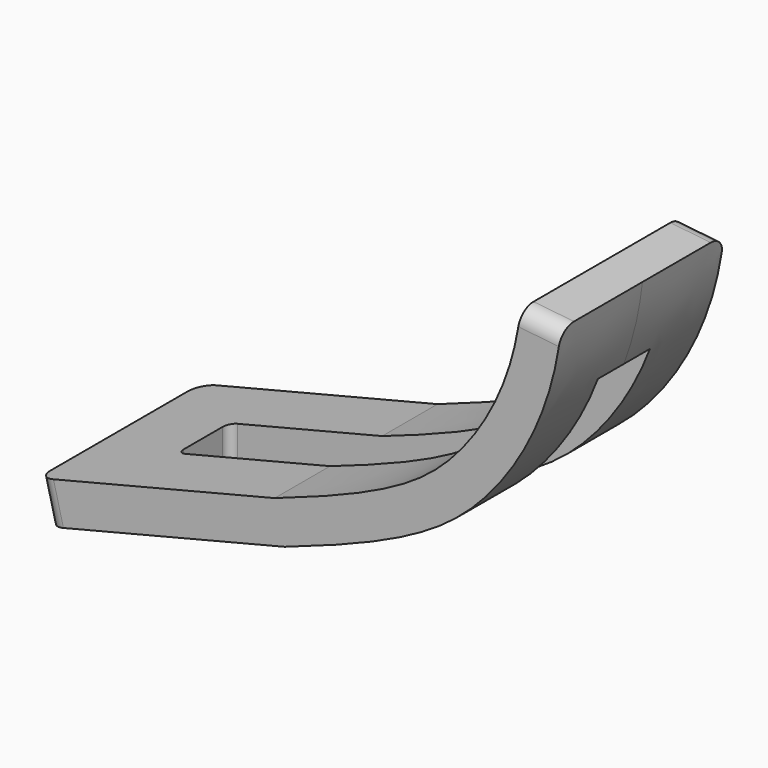
from build123d import *

# Parameters (mm, degrees)
F1_DEPTH      = 12.5
F1_DEPTH_BACK = 12.5
F2_R          = 2
F4_DEPTH      = 25
F4_DEPTH_BACK = 25


# Not quite as in the source:
# - ends of sketch curves that miss each other by under 0.0002 mm in the source are joined
# - the dataset's text gives a spline's control points without its knots; the knots are read off the source's solid


with BuildPart() as f1:
    # F0 (on Front) → F1 (new body, two sides)
    with BuildSketch(Plane.XZ) as f1_sk:
        with BuildLine():
            Line((-1.2184032821, 4.8688166534), (0, 0))
            add(Edge.make_bspline(
                [(0, 0), (13.9942302595, 4.8154504329), (25.3093838267, 10.870907846), (33.031907279, 25.9106602745), (33.9476719961, 34.5905660178)],
                knots=[0, 0, 0, 0, 0.5280763551, 1, 1, 1, 1], degree=3))
            Line((33.9476719961, 34.5905660178), (28.975269547, 35.1151743323))
            add(Edge.make_bspline(
                [(-1.2184032821, 4.8688166534), (1.8648217541, 5.9349029149), (7.287113618, 7.9315285829), (12.1983004489, 10.1724794599), (15.2865186932, 11.9439955294), (17.2413608312, 13.281183998), (18.9416466936, 14.6787902185), (20.2373870468, 15.9523435041), (21.2534611324, 17.0823993837), (22.2542990458, 18.283251609), (23.9332185037, 20.5443961427), (26.0676758341, 24.2225990158), (28.0070847052, 29.2983814533), (28.7632711893, 33.1057872835), (28.975269547, 35.1151743323)],
                knots=[0.0052558834, 0.0052558834, 0.0052558834, 0.0052558834, 0.125, 0.25, 0.3125, 0.375, 0.4375, 0.5, 0.53125, 0.5625, 0.625, 0.75, 0.875, 1, 1, 1, 1], degree=3))
        make_face()
        Polygon((-29.1025877416, -7.2828144797), (0, 0), (-1.2184032821, 4.8688166534), (-30.3209910237, -2.4139978263), align=None)
    extrude(amount=F1_DEPTH)
    extrude(f1_sk.sketch, amount=-F1_DEPTH_BACK)

    # F2
    f2_edges = [f1.edges().sort_by_distance(p)[0] for p in [
        (31.461471, -12.5, 34.85287),
        (31.461471, 12.5, 34.85287),
        (-29.711789, -12.5, -4.848406),
        (-29.711789, 12.5, -4.848406),
    ]]
    fillet(f2_edges, radius=F2_R)

    # F3 (on Top) → F4 (cut, two sides)
    with BuildSketch(Plane.XY) as f4_sk:
        with BuildLine():
            Line((-19, -4), (50, -4))
            Line((50, -4), (50, 4))
            Line((50, 4), (-19, 4))
            ThreePointArc((-19, 4), (-19.7071067812, 3.7071067812), (-20, 3))
            Line((-20, 3), (-20, -3))
            ThreePointArc((-20, -3), (-19.7071067812, -3.7071067812), (-19, -4))
        make_face()
    extrude(amount=F4_DEPTH, mode=Mode.SUBTRACT)
    extrude(f4_sk.sketch, amount=-F4_DEPTH_BACK, mode=Mode.SUBTRACT)


solid = f1.part
